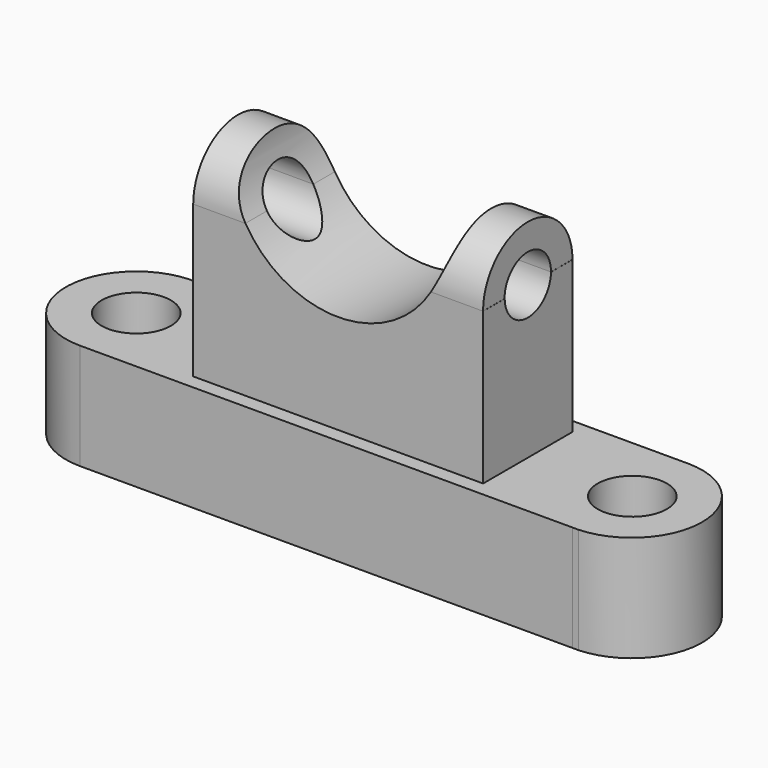
from build123d import *

# Parameters (mm, degrees)
F1_R      = 8.2936411115
F2_DEPTH  = 25.4
F3_W      = 69.4077983499
F3_H      = 26.76769346
F4_DEPTH  = 36.322
F7_DEPTH  = 69.3928
F8_DEPTH  = 100.584
F10_DEPTH = 29.464


with BuildPart() as f2:
    # F1 (on face) → F2 (new body)
    with BuildSketch(Plane.XY):
        with BuildLine():
            ThreePointArc((60.3076215597, -16.8506682543), (76.4416354881, 0.3672646239), (59.5732608546, 16.8664026399))
            Line((59.5732608546, 16.8664026399), (-57.860675973, 16.8248360129))
            ThreePointArc((-57.860675973, 16.8248360129), (-75.9001367339, 0.5909603363), (-59.041865465, -16.8664035499))
            Line((-59.041865465, -16.8664035499), (58.8552834129, -16.8508597338))
            Line((58.8552834129, -16.8508597338), (60.3076215597, -16.8506682543))
        make_face()
        with Locations((-59.0450726449, 0)):
            Circle(F1_R, mode=Mode.SUBTRACT)
        with Locations((59.7131252289, 0)):
            Circle(F1_R, mode=Mode.SUBTRACT)
    extrude(amount=F2_DEPTH)

    # F3 (on face) → F4 (join)
    with BuildSketch(Plane.XY.offset(25.4)):
        Rectangle(F3_W, F3_H)
    extrude(amount=F4_DEPTH)

    # F5 (on face) → F7 (join)
    with BuildSketch(Plane(origin=(-34.7038991749, 0, 0), x_dir=(0, -1, 0), z_dir=(-1, 0, 0))):
        with BuildLine():
            Line((-13.38384673, 61.722), (13.38384673, 61.722))
            ThreePointArc((13.38384673, 61.722), (0, 75.10584673), (-13.38384673, 61.722))
        make_face()
    extrude(amount=-F7_DEPTH)

    # F6 (on face) → F8 (cut)
    with BuildSketch(Plane(origin=(-34.7038991749, 0, 0), x_dir=(0, -1, 0), z_dir=(-1, 0, 0))):
        with BuildLine():
            Line((6.9332089114, 61.722), (-6.9332089114, 61.722))
            ThreePointArc((-6.9332089114, 61.722), (0, 54.9050340839), (6.9332089114, 61.722))
        make_face()
        with BuildLine():
            ThreePointArc((6.9332089114, 61.722), (6.9339522234, 61.7806149473), (6.9342, 61.8392340839))
            ThreePointArc((6.9342, 61.8392340839), (-0.0586191366, 68.7731863073), (-6.9332089114, 61.722))
            Line((-6.9332089114, 61.722), (6.9332089114, 61.722))
        make_face()
    extrude(amount=-F8_DEPTH, mode=Mode.SUBTRACT)

    # F9 (on face) → F10 (cut)
    with BuildSketch(Plane(origin=(0, 13.38384673, 0), x_dir=(-1, 0, 0), z_dir=(0, 1, 0))):
        with BuildLine():
            ThreePointArc((22.2074646178, 61.722), (24.9850855062, 68.1647563019), (25.9341114011, 75.116276741))
            ThreePointArc((25.9341114011, 75.116276741), (-6.9515204391, 100.1013622472), (-22.2074646178, 61.722))
            Line((-22.2074646178, 61.722), (22.2074646178, 61.722))
        make_face()
        with BuildLine():
            Line((22.2074646178, 61.722), (-22.2074646178, 61.722))
            ThreePointArc((-22.2074646178, 61.722), (0, 49.1821653399), (22.2074646178, 61.722))
        make_face()
    extrude(amount=-F10_DEPTH, mode=Mode.SUBTRACT)


solid = f2.part
